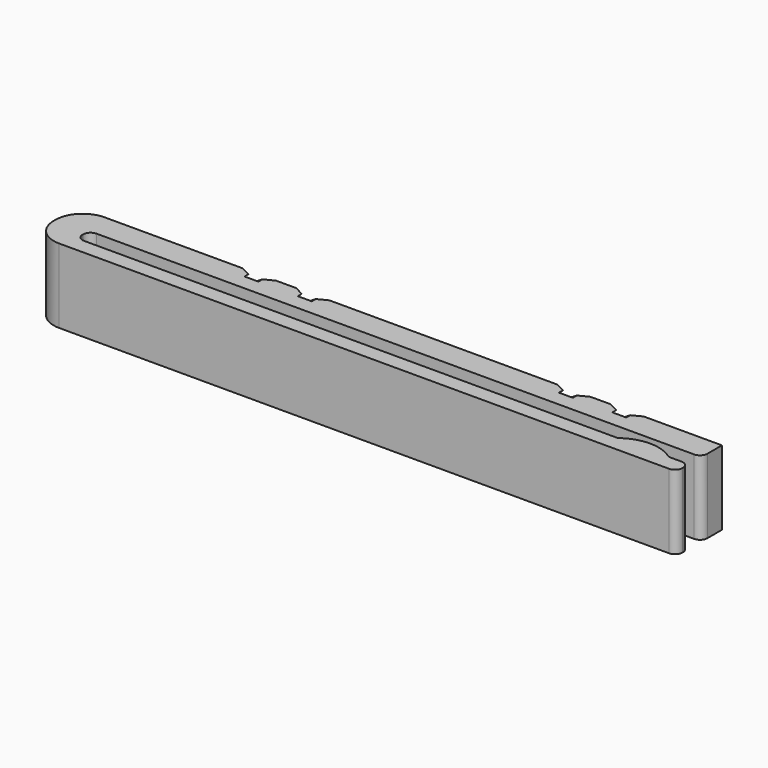
from build123d import *

# Parameters (mm, degrees)
F1_DEPTH    = 7.62
F3_DEPTH    = 1.016
F4_T1_DEPTH = 21.59
F5_R        = 0.762
F6_R        = 0.762
F7_SIZE     = 0.508


# Not quite as in the source:
# - a fillet or chamfer that OpenCascade refuses, or shapes differently, is made with other operations: its cross-section is extruded or revolved along the edge and cut away or added


with BuildPart() as f1:
    # F0 (on Top) → F1 (new body)
    with BuildSketch(Plane.XY):
        with BuildLine():
            Line((62.1792, 9.144), (-3.8608, 9.144))
            Line((-3.8608, 9.144), (-3.8608, 4.3472210688))
            Line((-3.8608, 4.3472210688), (62.1792, 4.3472210688))
            Line((62.1792, 4.3472210688), (62.1792, 5.9436))
            Line((62.1792, 5.9436), (60.087851236, 5.9436))
            ThreePointArc((60.087851236, 5.9436), (57.4883669615, 6.8209325844), (54.888882687, 5.9436))
            Line((54.888882687, 5.9436), (-0.5588, 5.9436))
            Line((-0.5588, 5.9436), (-0.5588, 7.5438))
            Line((-0.5588, 7.5438), (62.1792, 7.5438))
            Line((62.1792, 7.5438), (62.1792, 9.144))
        make_face()
    extrude(amount=F1_DEPTH)

    # F2 (on face) → F3 (join)
    with BuildSketch(Plane(origin=(0, 9.144, 0), x_dir=(-1, 0, 0), z_dir=(0, 1, 0))):
        Polygon((-14.0853170305, 7.62), (-1.3910392299, 0), (3.8608, 0), (3.8608, 7.62), align=None)
        Polygon((-19.5489563048, 7.62), (-6.8546785042, 0), (-2.8160745278, 0), (-15.5103523284, 7.62), align=None)
        Polygon((-33.6069809273, 0), (-8.279713802, 0), (-20.9739916027, 7.62), (-46.3012587279, 7.62), align=None)
        Polygon((-39.0706202015, 0), (-35.0320162252, 0), (-47.7262940258, 7.62), (-51.7648980021, 7.62), align=None)
        Polygon((-62.1792, 0), (-40.4956554994, 0), (-53.1899333, 7.62), (-62.1792, 7.62), align=None)
    extrude(amount=F3_DEPTH)

    # F4: fillet of radius 2.794 on 3 edges, made by hand

    # F4_s2 → F4_t1 (cut)
    with BuildSketch(Plane.XY.offset(-6.985)):
        with BuildLine():
            ThreePointArc((-1.0668, 4.3472210688), (-3.0424563466, 5.1655647222), (-3.8608, 7.1412210688))
            Line((-3.8608, 7.1412210688), (-3.8608, 4.3472210688))
            Line((-3.8608, 4.3472210688), (-1.0668, 4.3472210688))
        make_face()
        with BuildLine():
            ThreePointArc((-3.8608, 7.366), (-3.0424563466, 9.3416563466), (-1.0668, 10.16))
            Line((-1.0668, 10.16), (-3.8608, 10.16))
            Line((-3.8608, 10.16), (-3.8608, 7.366))
        make_face()
    extrude(amount=F4_T1_DEPTH, mode=Mode.SUBTRACT)

    # F5
    f5_edges = [f1.edges().sort_by_distance(p)[0] for p in [
        (-0.5588, 5.9436, 3.81),
        (-0.5588, 7.5438, 3.81),
    ]]
    fillet(f5_edges, radius=F5_R)

    # F6
    f6_edges = [f1.edges().sort_by_distance(p)[0] for p in [
        (62.1792, 7.5438, 3.81),
        (60.087851, 5.9436, 3.81),
        (62.1792, 5.9436, 3.81),
        (62.1792, 4.347221, 3.81),
    ]]
    fillet(f6_edges, radius=F6_R)

    # F7
    f7_edges = [f1.edges().sort_by_distance(p)[0] for p in [
        (7.738178, 10.16, 3.81),
        (9.163213, 10.16, 3.81),
        (13.201817, 10.16, 3.81),
        (14.626853, 10.16, 3.81),
        (39.95412, 10.16, 3.81),
        (41.379155, 10.16, 3.81),
        (45.417759, 10.16, 3.81),
        (46.842794, 10.16, 3.81),
    ]]
    chamfer(f7_edges, length=F7_SIZE)


solid = f1.part
